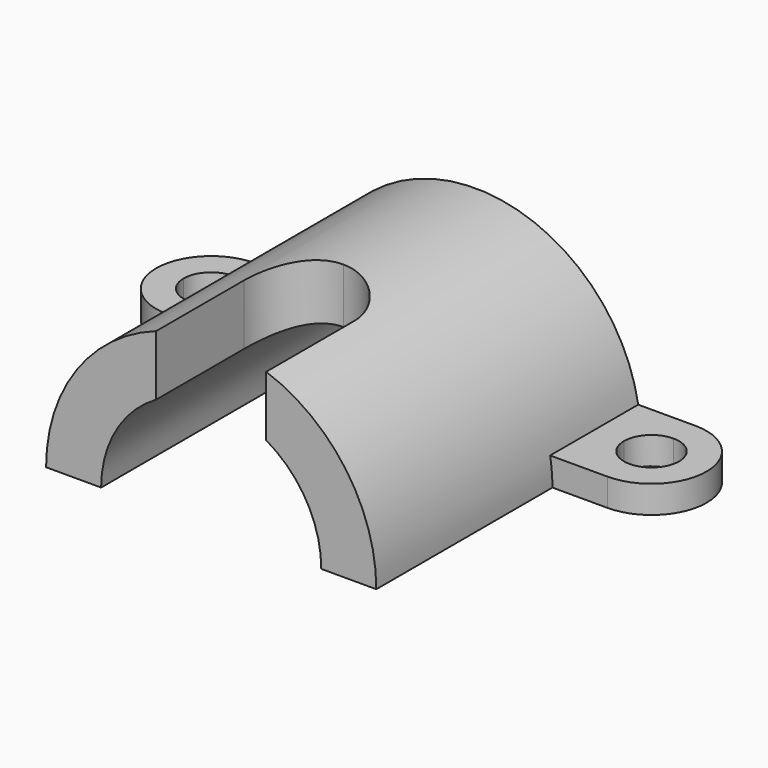
from build123d import *

# Parameters (mm, degrees)
F1_DEPTH  = 60
F3_DEPTH  = 5
F5_DEPTH  = 5.001
F7_DEPTH  = 5.001
F9_DEPTH  = 60.001
F11_REACH = 66.0565127546
F12_R     = 9.999


# Not quite as in the source:
# - a fillet or chamfer is up to 0.001 mm smaller than in the source, because OpenCascade refuses the exact size


with BuildPart() as f1:
    # F0 (on Front) → F1 (new body)
    with BuildSketch(Plane.XZ):
        with BuildLine():
            Line((-30, 0), (30, 0))
            ThreePointArc((30, 0), (0, 30), (-30, 0))
        make_face()
    extrude(amount=F1_DEPTH)

    # F2 (on face) → F3 (join)
    with BuildSketch(Plane(origin=(0, 0, 0), x_dir=(1, 0, 0), z_dir=(0, 0, -1))):
        with BuildLine():
            ThreePointArc((-40, 20), (-50, 10), (-40, 0))
            Line((-40, 0), (40, 0))
            ThreePointArc((40, 0), (50, 10), (40, 20))
            Line((40, 20), (-40, 20))
        make_face()
    extrude(amount=-F3_DEPTH)

    # F4 (on face) → F5 (cut, through all)
    with BuildSketch(Plane.XY.offset(5)):
        with BuildLine():
            Line((-45, -10), (-40, -10))
            Line((-40, -10), (-40, -5))
            ThreePointArc((-40, -5), (-43.5355339059, -6.4644660941), (-45, -10))
        make_face()
        with BuildLine():
            Line((-40, -5), (-40, -10))
            Line((-40, -10), (-35, -10))
            ThreePointArc((-35, -10), (-36.4644660941, -6.4644660941), (-40, -5))
        make_face()
        with BuildLine():
            Line((-40, -10), (-40, -15))
            ThreePointArc((-40, -15), (-36.4644660941, -13.5355339059), (-35, -10))
            Line((-35, -10), (-40, -10))
        make_face()
        with BuildLine():
            ThreePointArc((-45, -10), (-43.5355339059, -13.5355339059), (-40, -15))
            Line((-40, -15), (-40, -10))
            Line((-40, -10), (-45, -10))
        make_face()
    extrude(amount=-F5_DEPTH, mode=Mode.SUBTRACT)

    # F6 (on face) → F7 (cut, through all)
    with BuildSketch(Plane.XY.offset(5)):
        with BuildLine():
            ThreePointArc((40, -5), (36.4644660941, -6.4644660941), (35, -10))
            Line((35, -10), (40, -10))
            Line((40, -10), (40, -5))
        make_face()
        with BuildLine():
            Line((40, -5), (40, -10))
            Line((40, -10), (45, -10))
            ThreePointArc((45, -10), (43.5355339059, -6.4644660941), (40, -5))
        make_face()
        with BuildLine():
            Line((45, -10), (40, -10))
            Line((40, -10), (40, -15))
            ThreePointArc((40, -15), (43.5355339059, -13.5355339059), (45, -10))
        make_face()
        with BuildLine():
            Line((40, -10), (35, -10))
            ThreePointArc((35, -10), (36.4644660941, -13.5355339059), (40, -15))
            Line((40, -15), (40, -10))
        make_face()
    extrude(amount=-F7_DEPTH, mode=Mode.SUBTRACT)

    # F8 (on face) → F9 (cut, through all)
    with BuildSketch(Plane.XZ.offset(60)):
        with BuildLine():
            Line((-20, 0), (20, 0))
            ThreePointArc((20, 0), (0, 20), (-20, 0))
        make_face()
    extrude(amount=-F9_DEPTH, mode=Mode.SUBTRACT)

    f11_end = f1.faces().sort_by_distance((0, -30, 30))[0]
    # F10 (on Top) → F11 (cut, up to a face of the model that its end follows)
    with BuildSketch(Plane.XY):
        Polygon((-10, -60), (0, -60), (10, -60), (10, -30), (-10, -30), align=None)
    f11_long = extrude(amount=F11_REACH, mode=Mode.PRIVATE)
    add(split(f11_long, bisect_by=f11_end, keep=Keep.BOTTOM, mode=Mode.PRIVATE), mode=Mode.SUBTRACT)

    # F12 (radius 10 in the source; OpenCascade refuses exactly that, so slightly less here)
    f12_edges = [f1.edges().sort_by_distance(p)[0] for p in [
        (-10, -30, 22.80239),
        (10, -30, 22.80239),
    ]]
    fillet(f12_edges, radius=F12_R)


solid = f1.part
